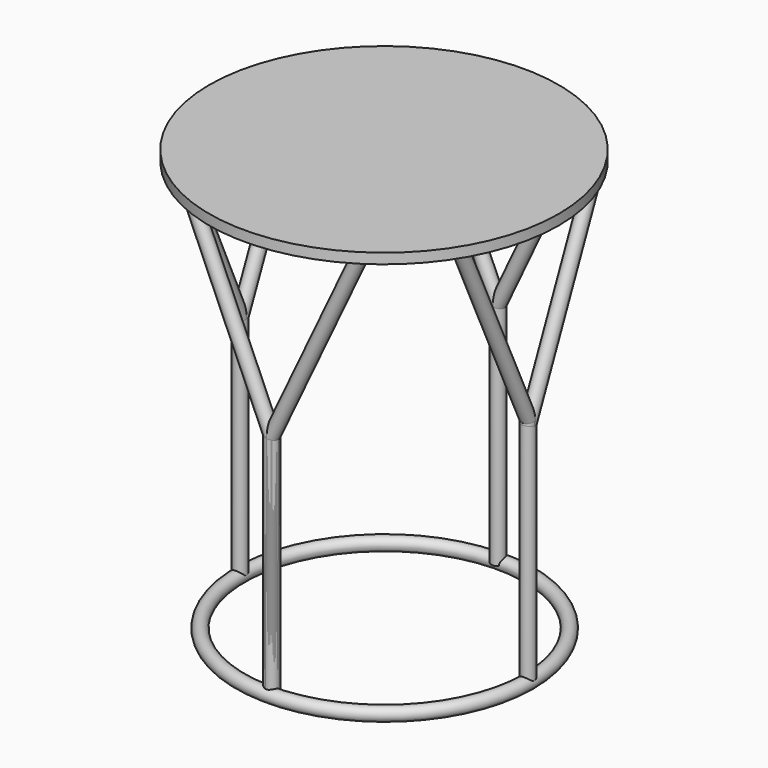
from build123d import *
from build123d import SkipClean  # not in build123d's __all__

# Parameters (mm, degrees)
F1_R     = 85
F2_DEPTH = 5
F3_R     = 3.2745059597
F17_R    = 3.274505
F16_R    = 3.274505
F15_R    = 3.274505
F27_R    = 3.275


with BuildPart() as f2:
    # F1 (on offset) → F2 (new body)
    with BuildSketch(Plane.XY.offset(200)):
        Circle(F1_R)
    extrude(amount=F2_DEPTH)

    # F18: sweep along a path in F11
    with BuildLine(Plane.YZ.offset(-70)) as f18_path:
        Line((0, 0), (0, 110.7534617186))
        Line((0, 110.7534617186), (40.7959488519, 202.7134001255))
    # F17 (on Top) → F18 (sweep)
    with BuildSketch(Plane.XY):
        with Locations((-70.0240433216, 0)):
            Circle(F17_R)
    sweep(path=f18_path.line, transition=Transition.RIGHT)

    # F20: sweep along a path in F19
    with BuildLine(Plane.YZ.offset(-70)) as f20_path:
        Line((0, 0), (0, 110.7534617186))
        Line((0, 110.7534617186), (-40.5439175665, 201.8073946238))
    # F17 (on Top) → F20 (sweep)
    with BuildSketch(Plane.XY):
        with Locations((-70.0240433216, 0)):
            Circle(F17_R)
    sweep(path=f20_path.line, transition=Transition.RIGHT)

    # F21: sweep along a path in F9
    with BuildLine(Plane.YZ.offset(70)) as f21_path:
        Line((0, 0), (0, 110.3004589677))
        Line((0, 110.3004589677), (40.0909073651, 201.8073946238))
    # F16 (on Top) → F21 (sweep)
    with BuildSketch(Plane.XY):
        with Locations((70.058837533, 0)):
            Circle(F16_R)
    sweep(path=f21_path.line, transition=Transition.RIGHT)

    # F23: sweep along a path in F22
    with BuildLine(Plane.YZ.offset(70)) as f23_path:
        Line((0, 0), (0, 112.5654801726))
        Line((0, 112.5654801726), (-41.9029258192, 203.166410327))
    # F16 (on Top) → F23 (sweep)
    with BuildSketch(Plane.XY):
        with Locations((70.058837533, 0)):
            Circle(F16_R)
    with SkipClean():  # cleaning this boolean's faces spoils the solid; the shape is the same uncleaned
        sweep(path=f23_path.line, transition=Transition.RIGHT)

    # F25: sweep along a path in F10
    with BuildLine(Plane.XZ.offset(-70)) as f25_path:
        Line((0, 0), (0, 110.7534617186))
        Line((0, 110.7534617186), (42.8089387715, 201.8073946238))
    # F15 (on Top) → F25 (sweep)
    with BuildSketch(Plane.XY):
        with Locations((0, 69.3760632882)):
            Circle(F15_R)
    with SkipClean():  # cleaning this boolean's faces spoils the solid; the shape is the same uncleaned
        sweep(path=f25_path.line, transition=Transition.RIGHT)

    # F26: sweep along a path in F24
    with BuildLine(Plane.XZ.offset(-70)) as f26_path:
        Line((0, 0), (0, 110.7534617186))
        Line((0, 110.7534617186), (-40.9969165921, 203.166410327))
    # F15 (on Top) → F26 (sweep)
    with BuildSketch(Plane.XY):
        with Locations((0, 69.3760632882)):
            Circle(F15_R)
    with SkipClean():  # cleaning this boolean's faces spoils the solid; the shape is the same uncleaned
        sweep(path=f26_path.line, transition=Transition.RIGHT)


with BuildPart() as f12:
    # F12: sweep along a path in F5
    with BuildLine(Plane.XZ.offset(70)) as f12_path:
        Line((0, 0), (0, 110.3004589677))
        Line((0, 110.3004589677), (43.5006563944, 202.260389924))
    # F3 (on Top) → F12 (sweep)
    with BuildSketch(Plane.XY):
        with Locations((0, -68.2542175055)):
            Circle(F3_R)
    sweep(path=f12_path.line, transition=Transition.RIGHT)


with BuildPart() as f14:
    # F14: sweep along a path in F13
    with BuildLine(Plane.XZ.offset(70)) as f14_path:
        Line((0, 0), (0, 110.7534617186))
        Line((0, 110.7534617186), (-39.6379046142, 201.3543844223))
    # F3 (on Top) → F14 (sweep)
    with BuildSketch(Plane.XY):
        with Locations((0, -68.2542175055)):
            Circle(F3_R)
    sweep(path=f14_path.line, transition=Transition.RIGHT)


with BuildPart() as f29:
    # F29: sweep along a path in F28
    with BuildLine(Plane.XY) as f29_path:
        CenterArc((0.1617685287, 0.2007872436), 67.5, 0, 360)
    # F27 (on Front) → F29 (sweep)
    with BuildSketch(Plane.XZ):
        with Locations((-70.0292140245, 0)):
            Circle(F27_R)
    sweep(path=f29_path.line)


solid = Compound([f2.part, f12.part, f14.part, f29.part])
